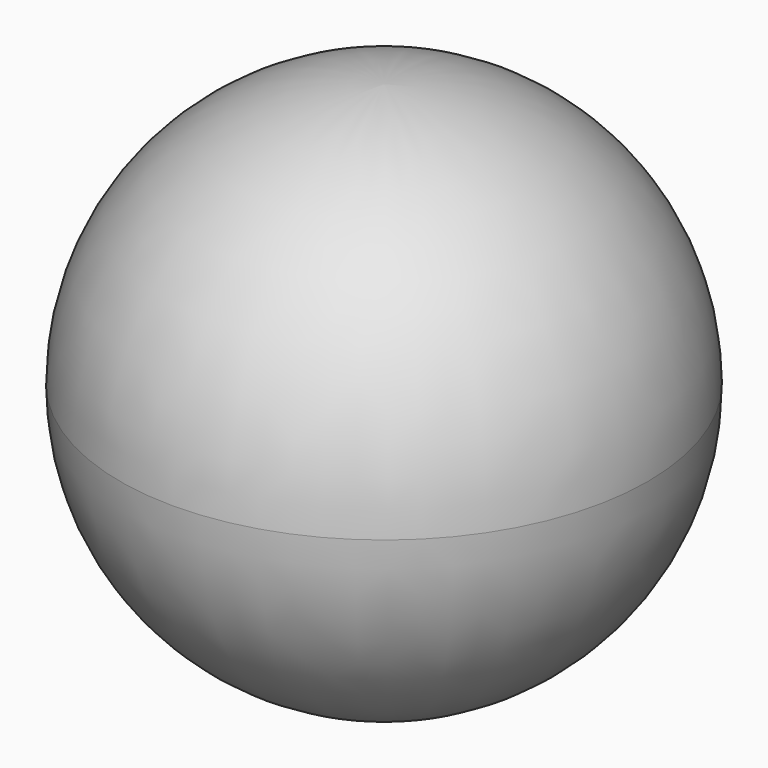
from build123d import *

# Parameters (mm, degrees)
F0_R     = 37.5
F1_DEPTH = 37.5
F2_R     = 37.49999


# Not quite as in the source:
# - a fillet or chamfer is up to 0.001 mm smaller than in the source, because OpenCascade refuses the exact size


with BuildPart() as f1:
    # F0 (on Top) → F1 (new body, symmetric)
    with BuildSketch(Plane.XY):
        Circle(F0_R)
    extrude(amount=F1_DEPTH, both=True)

    # F2 (radius 37.5 in the source; OpenCascade refuses exactly that, so slightly less here)
    f2_edges = [f1.edges().sort_by_distance(p)[0] for p in [
        (-37.5, 0, 37.5),
        (-37.5, 0, -37.5),
    ]]
    fillet(f2_edges, radius=F2_R)


solid = f1.part
